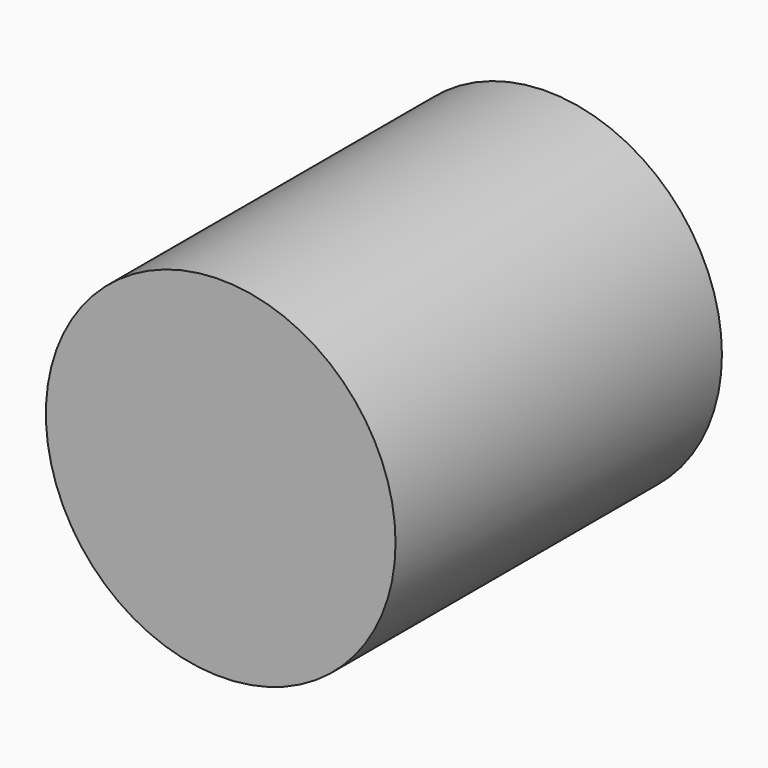
from build123d import *

# Parameters (mm, degrees)
F1_R     = 76.2
F2_DEPTH = 177.8


# Not quite as in the source:
# - a variable given as a bare number and used for a length is read in inches; the dataset says mm whatever the document's units were


with BuildPart() as f2:
    # F1 (on Front) → F2 (new body)
    with BuildSketch(Plane.XZ):
        Circle(F1_R)
    extrude(amount=F2_DEPTH)


solid = f2.part
